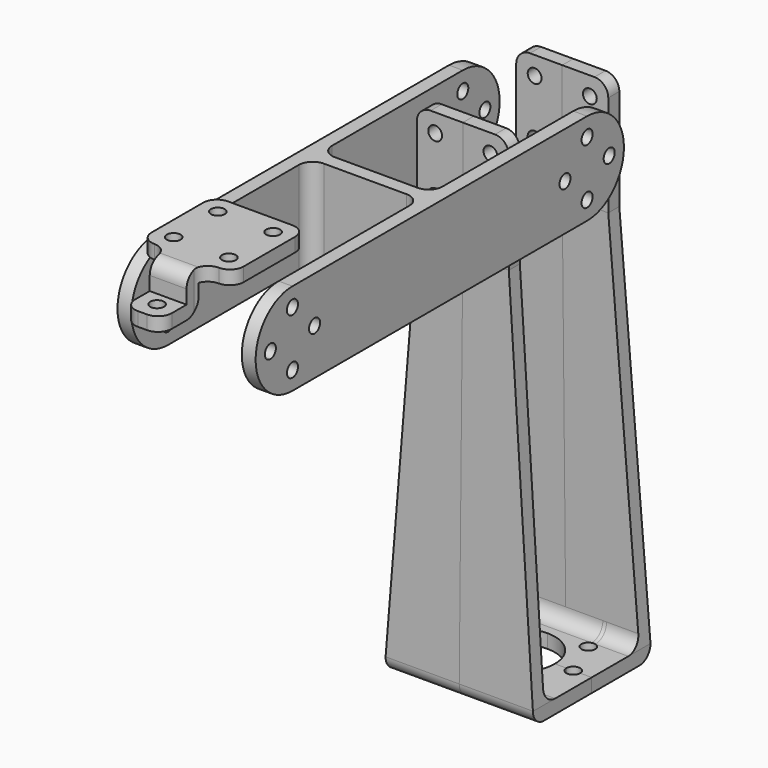
from build123d import *
from build123d import SkipClean  # not in build123d's __all__

# Parameters (mm, degrees)
F6_DEPTH  = 16
F7_R      = 1.5
F8_DEPTH  = 16.001
F9_R      = 1.5
F9_R_2    = 8
F10_DEPTH = 3
F11_R     = 3
F14_R     = 1.5
F15_DEPTH = 15
F17_START = 25
F17_DEPTH = 50
F20_DEPTH = 10
F21_R     = 1.5
F22_DEPTH = 25
F23_R     = 2.99999


# Not quite as in the source:
# - a fillet or chamfer is up to 0.001 mm smaller than in the source, because OpenCascade refuses the exact size


with BuildPart() as f6:
    # F5 (on Right) → F6 (new body)
    with BuildSketch(Plane.YZ):
        Polygon((0, 0), (0, 3), (-12.9647058824, 3), (-12, 85), (-12, 110), (-15, 110), (-15, 85), (-16, 0), align=None)
    extrude(amount=F6_DEPTH)

    # F7 (on Front) → F8 (cut, through all)
    with BuildSketch(Plane.XZ):
        Polygon((16, 110), (10, 110), (10, 85), (16, 3), align=None)
        with Locations((6, 106)):
            Circle(F7_R)
        with Locations((6, 94)):
            Circle(F7_R)
    extrude(amount=F8_DEPTH, mode=Mode.SUBTRACT)

    # F9 (on Top) → F10 (cut, through all)
    with BuildSketch(Plane.XY):
        with Locations((12, 0)):
            Circle(F9_R)
        with Locations((8.4852813742, -8.4852813742)):
            Circle(F9_R)
        Circle(F9_R_2)
    extrude(amount=F10_DEPTH, mode=Mode.SUBTRACT)

    # F11
    f11_edges = [f6.edges().sort_by_distance(p)[0] for p in [
        (10, -13.5, 110),
        (8, -16, 0),
        (8, -12.964706, 3),
    ]]
    fillet(f11_edges, radius=F11_R)

    # F12: F6 across plane


with BuildPart() as f6_1:
    add(f6.part, clean=False)
    add(f6.part.mirror(Plane.YZ), clean=False)

    # F13: F6 across plane


with BuildPart() as f6_2:
    add(f6_1.part, clean=False)
    with SkipClean():  # cleaning this boolean's faces spoils the solid; the shape is the same uncleaned
        add(f6_1.part.mirror(Plane.XZ), clean=False)


with BuildPart() as f15:
    # F14 (on Right) → F15 (new body)
    with BuildSketch(Plane.YZ):
        with BuildLine():
            ThreePointArc((-80, 110), (-90, 100), (-80, 90))
            Line((-80, 90), (0, 90))
            ThreePointArc((0, 90), (10, 100), (0, 110))
            Line((0, 110), (-80, 110))
        make_face()
        with Locations((-80, 94)):
            Circle(F14_R, mode=Mode.SUBTRACT)
        with Locations((0, 94)):
            Circle(F14_R, mode=Mode.SUBTRACT)
        with Locations((-86, 100)):
            Circle(F14_R, mode=Mode.SUBTRACT)
        with Locations((-74, 100)):
            Circle(F14_R, mode=Mode.SUBTRACT)
        with Locations((-80, 106)):
            Circle(F14_R, mode=Mode.SUBTRACT)
        with Locations((-6, 100)):
            Circle(F14_R, mode=Mode.SUBTRACT)
        with Locations((6, 100)):
            Circle(F14_R, mode=Mode.SUBTRACT)
        with Locations((0, 106)):
            Circle(F14_R, mode=Mode.SUBTRACT)
    extrude(amount=F15_DEPTH)

    # F16 (on plane+point) → F17 (intersect)
    with BuildSketch(Plane.XY.offset(100).offset(F17_START)):
        with BuildLine():
            Line((12, -90), (15, -90))
            Line((15, -90), (15, 10))
            Line((15, 10), (12, 10))
            Line((12, 10), (12, -35.5))
            ThreePointArc((12, -35.5), (11.1213203436, -37.6213203436), (9, -38.5))
            Line((9, -38.5), (0, -38.5))
            Line((0, -38.5), (0, -41.5))
            Line((0, -41.5), (9, -41.5))
            ThreePointArc((9, -41.5), (11.1213203436, -42.3786796564), (12, -44.5))
            Line((12, -44.5), (12, -90))
        make_face()
    extrude(amount=-F17_DEPTH, mode=Mode.INTERSECT)

    # F18: F15 across plane


with BuildPart() as f15_1:
    add(f15.part, clean=False)
    add(f15.part.mirror(Plane.YZ), clean=False)


with BuildPart() as f20:
    # F19 (on Right) → F20 (new body)
    with BuildSketch(Plane.YZ):
        with BuildLine():
            Line((-95, 112), (-95, 109))
            Line((-95, 109), (-102, 109))
            Line((-102, 109), (-102, 106))
            Line((-102, 106), (-95, 106))
            ThreePointArc((-95, 106), (-92.8786796564, 106.8786796564), (-92, 109))
            Line((-92, 109), (-92, 112))
            Line((-92, 112), (-70, 112))
            Line((-70, 112), (-70, 115))
            Line((-70, 115), (-92, 115))
            ThreePointArc((-92, 115), (-94.1213203436, 114.1213203436), (-95, 112))
        make_face()
    extrude(amount=F20_DEPTH)

    # F21 (on plane+point) → F22 (cut)
    with BuildSketch(Plane.XY.offset(100)):
        with Locations((0, -98)):
            Circle(F21_R)
        with Locations((6, -86)):
            Circle(F21_R)
        with Locations((6, -74)):
            Circle(F21_R)
        with BuildLine():
            Line((4, -93), (4, -102))
            Line((4, -102), (10, -102))
            Line((10, -102), (10, -90))
            Line((10, -90), (7, -90))
            ThreePointArc((7, -90), (4.8786796564, -90.8786796564), (4, -93))
        make_face()
    extrude(amount=F22_DEPTH, mode=Mode.SUBTRACT)

    # F23 (radius 3 in the source; OpenCascade refuses exactly that, so slightly less here)
    f23_edges = [f20.edges().sort_by_distance(p)[0] for p in [
        (10, -90, 113.5),
        (10, -70, 113.5),
        (4, -102, 107.5),
    ]]
    fillet(f23_edges, radius=F23_R)

    # F24: F20 across plane


with BuildPart() as f20_1:
    add(f20.part, clean=False)
    add(f20.part.mirror(Plane.YZ), clean=False)


solid = Compound([f6_2.part, f15_1.part, f20_1.part])
